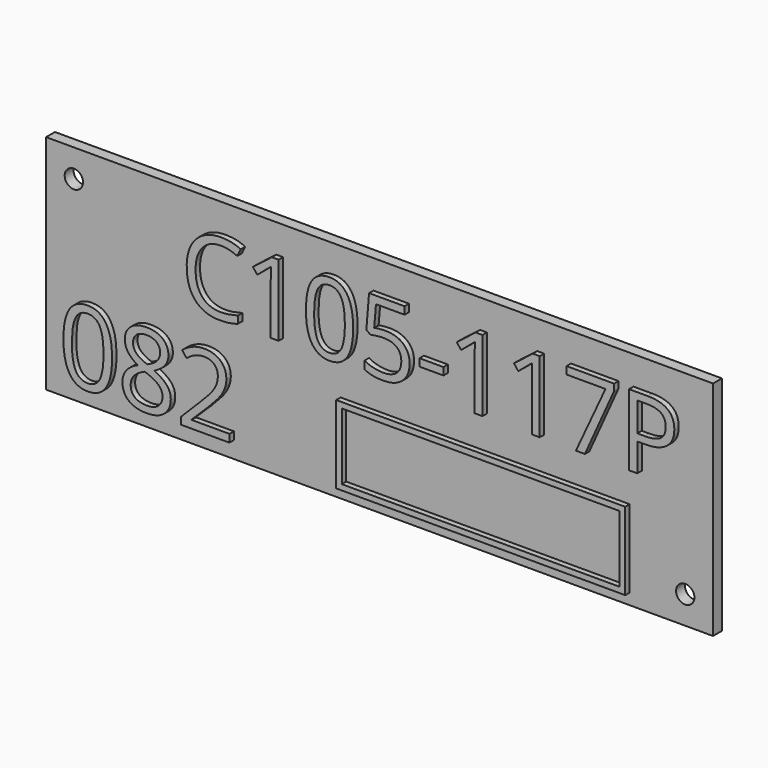
from build123d import *

# Parameters (mm, degrees)
F0_W         = 120
F0_H         = 40
F1_DEPTH     = 2
F3_D         = 3.3
F4_TEXT_SIZE = 18.0050639242
F5_DEPTH     = 1
F6_TEXT_SIZE = 18.5356140827
F7_DEPTH     = 1
F8_W         = 52
F8_H         = 14
F8_W_2       = 49.99999962
F8_H_2       = 11.99999962
F9_DEPTH     = 1


# Not quite as in the source:
# - Text() gives the source's letters only with a copy of the font that has no kerning and outlines rounded to 1/6400 em; it was checked with that copy


with BuildPart() as f1:
    # F0 (on Front) → F1 (new body)
    with BuildSketch(Plane.XZ):
        Rectangle(F0_W, F0_H)
    extrude(amount=F1_DEPTH)

    # F3 (through all)
    with Locations(Plane.XZ.offset(2)):
        with Locations((-55, 15), (55, -15)):
            Hole(F3_D / 2)

    # F4 (on face) → F5 (join)
    with BuildSketch(Plane.XZ.offset(2)):
        with Locations((-35, 2)):
            Text('C105-117P', F4_TEXT_SIZE, font='Open Sans', text_align=(TextAlign.LEFT, TextAlign.BOTTOM))
    extrude(amount=F5_DEPTH)

    # F6 (on face) → F7 (join)
    with BuildSketch(Plane.XZ.offset(2)):
        with Locations((-57, -17)):
            Text('082', F6_TEXT_SIZE, font='Open Sans', text_align=(TextAlign.LEFT, TextAlign.BOTTOM))
    extrude(amount=F7_DEPTH)

    # F8 (on face) → F9 (join)
    with BuildSketch(Plane.XZ.offset(2)):
        with Locations((19, -11)):
            Rectangle(F8_W, F8_H)
        with Locations((19, -11)):
            Rectangle(F8_W_2, F8_H_2, mode=Mode.SUBTRACT)
    extrude(amount=F9_DEPTH)


solid = f1.part
